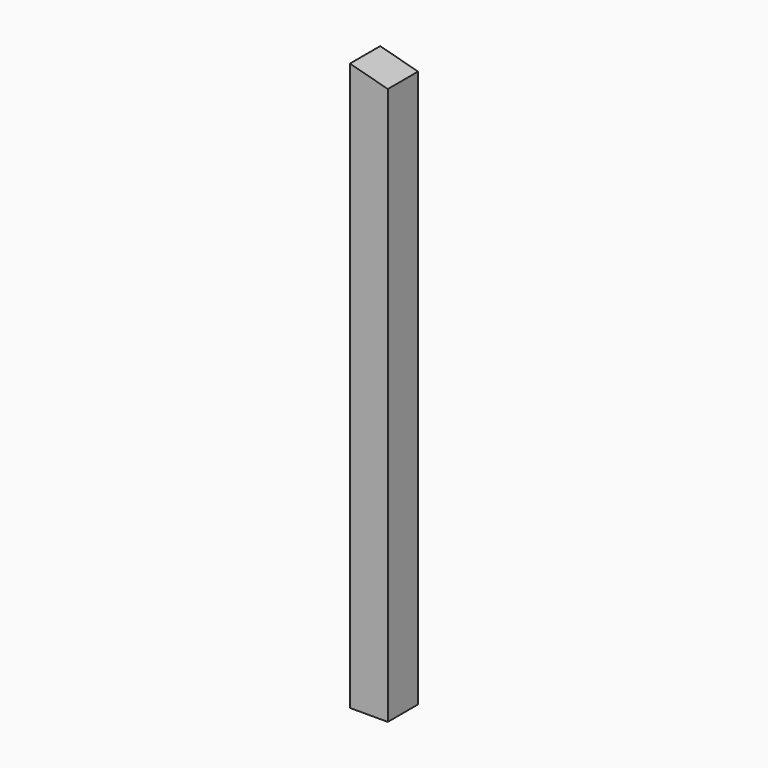
from build123d import *

# Parameters (mm, degrees)
F0_W     = 75
F0_H     = 75
F1_DEPTH = 1125
F2_SIZE2 = 20.096179
F2_SIZE  = 74.99999


# Not quite as in the source:
# - a fillet or chamfer is up to 0.001 mm smaller than in the source, because OpenCascade refuses the exact size


with BuildPart() as f1:
    # F0 (on Top) → F1 (new body)
    with BuildSketch(Plane.XY):
        Rectangle(F0_W, F0_H)
    extrude(amount=F1_DEPTH)

    # F2 (size 75 and 20.0961894323 in the source; OpenCascade refuses exactly that, so slightly less here)
    f2_edges = [f1.edges().sort_by_distance(p)[0] for p in [
        (37.5, 0, 1125),
    ]]
    f2_side = f1.faces().sort_by_distance((0, 0, 1125))[0]
    chamfer(f2_edges, length=F2_SIZE, length2=F2_SIZE2, reference=f2_side)


solid = f1.part
